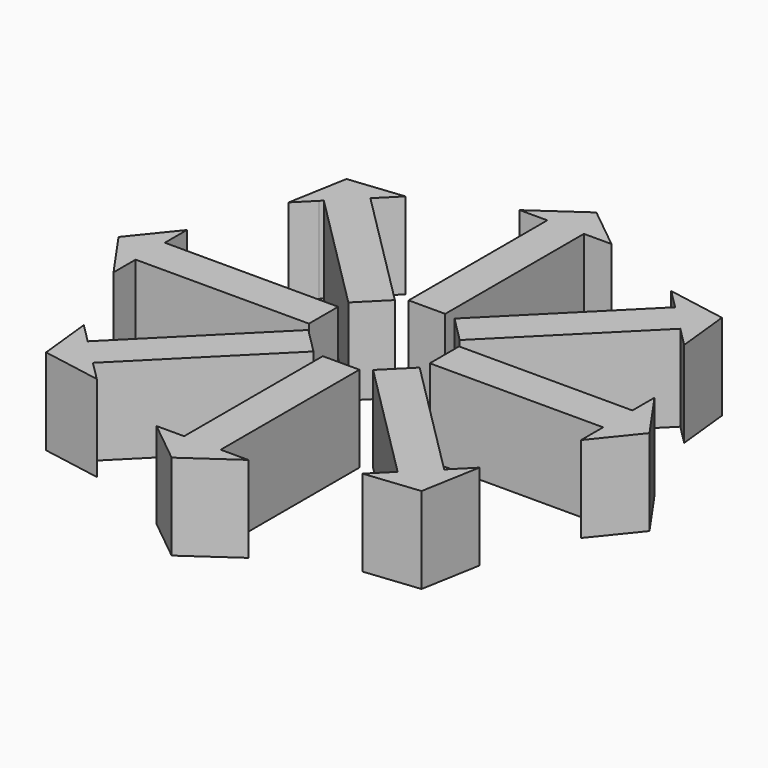
from build123d import *

# Parameters (mm, degrees)
F1_DEPTH = 0.5


# Not quite as in the source:
# - a feature names something its author has since deleted; it is built from what else it names


with BuildPart() as f1:
    # F0 (on Top) → F1 (new body)
    with BuildSketch(Plane.XY):
        Polygon((-1.3399171252, 0.0368332625), (-1.3399171252, -0.0368332625), (-1.3399171252, -0.125143673), (-0.3350383195, -0.125143673), (-0.3350383195, -0.0368332625), (-0.3350383195, 0.0368332625), (-0.3350383195, 0.0868332625), (-1.3399171252, 0.0868332625), align=None)
        Polygon((-1.3399171252, -0.125143673), (-1.3399171252, -0.0368332625), (-1.3399171252, 0.0368332625), (-1.3399171252, 0.0868332625), (-1.3399171252, 0.14733305), (-1.3399171252, 0.2468332625), (-1.5391977504, 0), (-1.3399171252, -0.285143673), (-1.3399171252, -0.14733305), align=None)
    extrude(amount=F1_DEPTH)


with BuildPart() as f1b:
    # F0 (on Top) → F1, piece 2 (new body)
    with BuildSketch(Plane.XY):
        Polygon((-0.1755074789, 0.2983082564), (-0.8860640967, 1.0088648742), (-0.9214194358, 0.9735095352), (-0.9735095352, 0.9214194358), (-1.0359544253, 0.8589745457), (-0.3253978074, 0.1484179279), (-0.2629529173, 0.210862818), (-0.210862818, 0.2629529173), align=None)
        Polygon((-0.9214194358, 0.9735095352), (-0.8860640967, 1.0088648742), (-0.8432842867, 1.0516446842), (-0.7729270117, 1.1220019592), (-1.0883771669, 1.0883771669), (-1.1490915102, 0.7458374607), (-1.0516446842, 0.8432842867), (-1.0359544253, 0.8589745457), (-0.9735095352, 0.9214194358), align=None)
    extrude(amount=F1_DEPTH)


with BuildPart() as f1c:
    # F0 (on Top) → F1, piece 3 (new body)
    with BuildSketch(Plane.XY):
        Polygon((0.0368332625, 1.3399171252), (0.0868332625, 1.3399171252), (0.14733305, 1.3399171252), (0.2468332625, 1.3399171252), (0, 1.5391977504), (-0.285143673, 1.3399171252), (-0.14733305, 1.3399171252), (-0.125143673, 1.3399171252), (-0.0368332625, 1.3399171252), align=None)
        Polygon((0.0868332625, 0.3350383195), (0.0868332625, 1.3399171252), (0.0368332625, 1.3399171252), (-0.0368332625, 1.3399171252), (-0.125143673, 1.3399171252), (-0.125143673, 0.3350383195), (-0.0368332625, 0.3350383195), (0.0368332625, 0.3350383195), align=None)
    extrude(amount=F1_DEPTH)


with BuildPart() as f1d:
    # F0 (on Top) → F1, piece 4 (new body)
    with BuildSketch(Plane.XY):
        Polygon((0.2983082564, 0.1755074789), (1.0088648742, 0.8860640967), (0.9735095352, 0.9214194358), (0.9214194358, 0.9735095352), (0.8589745457, 1.0359544253), (0.1484179279, 0.3253978074), (0.210862818, 0.2629529173), (0.2629529173, 0.210862818), align=None)
        Polygon((0.9735095352, 0.9214194358), (1.0088648742, 0.8860640967), (1.0516446842, 0.8432842867), (1.1220019592, 0.7729270117), (1.0883771669, 1.0883771669), (0.7458374607, 1.1490915102), (0.8432842867, 1.0516446842), (0.8589745457, 1.0359544253), (0.9214194358, 0.9735095352), align=None)
    extrude(amount=F1_DEPTH)


with BuildPart() as f1e:
    # F0 (on Top) → F1, piece 5 (new body)
    with BuildSketch(Plane.XY):
        Polygon((1.3399171252, -0.0368332625), (1.3399171252, -0.0868332625), (1.3399171252, -0.14733305), (1.3399171252, -0.2468332625), (1.5391977504, 0), (1.3399171252, 0.285143673), (1.3399171252, 0.14733305), (1.3399171252, 0.125143673), (1.3399171252, 0.0368332625), align=None)
        Polygon((0.3350383195, -0.0868332625), (1.3399171252, -0.0868332625), (1.3399171252, -0.0368332625), (1.3399171252, 0.0368332625), (1.3399171252, 0.125143673), (0.3350383195, 0.125143673), (0.3350383195, 0.0368332625), (0.3350383195, -0.0368332625), align=None)
    extrude(amount=F1_DEPTH)


with BuildPart() as f1f:
    # F0 (on Top) → F1, piece 6 (new body)
    with BuildSketch(Plane.XY):
        Polygon((0.1755074789, -0.2983082564), (0.8860640967, -1.0088648742), (0.9214194358, -0.9735095352), (0.9735095352, -0.9214194358), (1.0359544253, -0.8589745457), (0.3253978074, -0.1484179279), (0.2629529173, -0.210862818), (0.210862818, -0.2629529173), align=None)
        Polygon((0.9214194358, -0.9735095352), (0.8860640967, -1.0088648742), (0.8432842867, -1.0516446842), (0.7729270117, -1.1220019592), (1.0883771669, -1.0883771669), (1.1490915102, -0.7458374607), (1.0516446842, -0.8432842867), (1.0359544253, -0.8589745457), (0.9735095352, -0.9214194358), align=None)
    extrude(amount=F1_DEPTH)


with BuildPart() as f1g:
    # F0 (on Top) → F1, piece 7 (new body)
    with BuildSketch(Plane.XY):
        Polygon((-0.0868332625, -0.3350383195), (-0.0868332625, -1.3399171252), (-0.0368332625, -1.3399171252), (0.0368332625, -1.3399171252), (0.125143673, -1.3399171252), (0.125143673, -0.3350383195), (0.0368332625, -0.3350383195), (-0.0368332625, -0.3350383195), align=None)
        Polygon((-0.14733305, -1.3399171252), (-0.2468332625, -1.3399171252), (0, -1.5391977504), (0.285143673, -1.3399171252), (0.14733305, -1.3399171252), (0.125143673, -1.3399171252), (0.0368332625, -1.3399171252), (-0.0368332625, -1.3399171252), (-0.0868332625, -1.3399171252), align=None)
    extrude(amount=F1_DEPTH)


with BuildPart() as f1h:
    # F0 (on Top) → F1, piece 8 (new body)
    with BuildSketch(Plane.XY):
        Polygon((-1.0516446842, -0.8432842867), (-1.1220019592, -0.7729270117), (-1.0883771669, -1.0883771669), (-0.7458374607, -1.1490915102), (-0.8432842867, -1.0516446842), (-0.8589745457, -1.0359544253), (-0.9214194358, -0.9735095352), (-0.9735095352, -0.9214194358), (-1.0088648742, -0.8860640967), align=None)
        Polygon((-0.2983082564, -0.1755074789), (-1.0088648742, -0.8860640967), (-0.9735095352, -0.9214194358), (-0.9214194358, -0.9735095352), (-0.8589745457, -1.0359544253), (-0.1484179279, -0.3253978074), (-0.210862818, -0.2629529173), (-0.2629529173, -0.210862818), align=None)
    extrude(amount=F1_DEPTH)


solid = Compound([f1.part, f1b.part, f1c.part, f1d.part, f1e.part, f1f.part, f1g.part, f1h.part])
